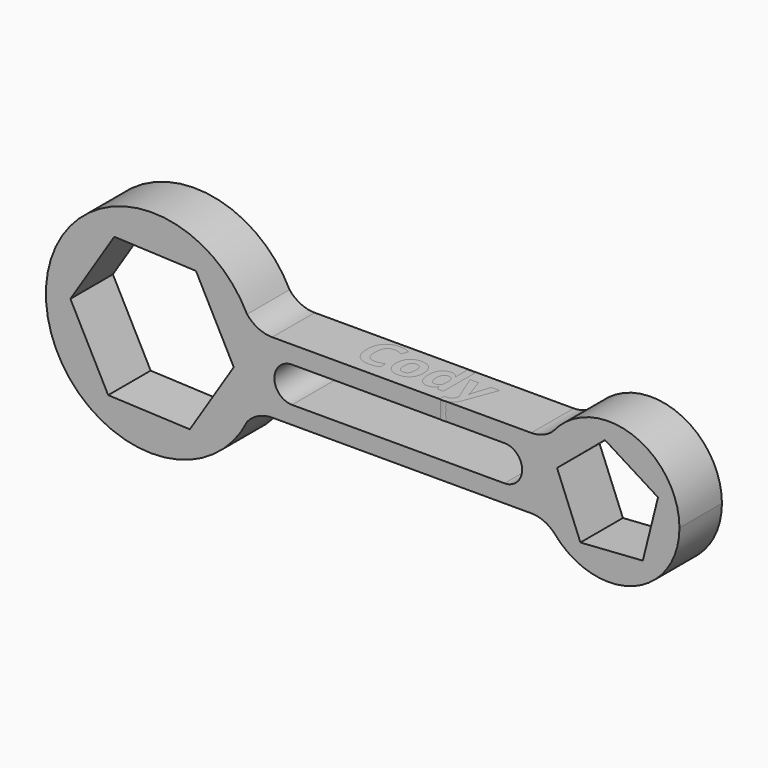
from build123d import *

# Parameters (mm, degrees)
F1_DEPTH     = 15
F2_TEXT_SIZE = 14.6601352349
F3_DEPTH     = 5


# Not quite as in the source:
# - Text() gives the source's letters only with a copy of the font that has no kerning and outlines rounded to 1/6400 em; it was checked with that copy


with BuildPart() as f1:
    # F0 (on Front) → F1 (new body)
    with BuildSketch(Plane.XZ):
        with BuildLine():
            ThreePointArc((-44.5868543681, -13.2794933275), (-42.2727545329, -6.8181696844), (-41.4876918451, 0))
            ThreePointArc((-41.4876918451, 0), (-42.2876779784, 6.8818013765), (-44.6449711908, 13.3965797082))
            ThreePointArc((-44.6449711908, 13.3965797082), (-101.4876206501, -0.065358216), (-44.5868543681, -13.2794933275))
        make_face()
        Polygon((-60.8156703444, -20.4802658777), (-83.8881116211, -19.4823746682), (-94.5601331218, 0.9978912095), (-82.1597133458, 20.4802658777), (-59.0872720691, 19.4823746682), (-48.4152505684, -0.9978912095), align=None, mode=Mode.SUBTRACT)
        with BuildLine():
            ThreePointArc((41.9423593748, 12.5529556275), (37.5154482696, -0.3543934672), (42.3969355922, -13.0967748813))
            ThreePointArc((42.3969355922, -13.0967748813), (64.5013191274, -18.7390961796), (77.5123081549, 0))
            ThreePointArc((77.5123081549, 0), (64.1681711492, 18.8599970255), (41.9423593748, 12.5529556275))
        make_face()
        Polygon((42.9262094907, 3.6496239321), (56.4759544087, 15), (71.4579049796, 5.6208858991), (67.1675147321, -11.5261014675), (49.5339571634, -12.7444083638), align=None, mode=Mode.SUBTRACT)
        with BuildLine():
            ThreePointArc((-44.6449711908, 13.3965797082), (-42.2876779784, 6.8818013765), (-41.4876918451, 0))
            ThreePointArc((-41.4876918451, 0), (-42.2727545329, -6.8181696844), (-44.5868543681, -13.2794933275))
            ThreePointArc((-44.5868543681, -13.2794933275), (-41.4324995346, -10.8601417529), (-37.551343441, -10))
            Line((-37.551343441, -10), (35.6224104762, -10))
            ThreePointArc((35.6224104762, -10), (39.3467965066, -10.8108939133), (42.3969355922, -13.0967748813))
            ThreePointArc((42.3969355922, -13.0967748813), (37.5154482696, -0.3543934672), (41.9423593748, 12.5529556275))
            ThreePointArc((41.9423593748, 12.5529556275), (39.0304647788, 10.6623457158), (35.6224104762, 10))
            Line((35.6224104762, 10), (-37.551343441, 10))
            ThreePointArc((-37.551343441, 10), (-41.4837825177, 10.8929262627), (-44.6449711908, 13.3965797082))
        make_face()
        with BuildLine():
            ThreePointArc((-31.9349189311, -5), (-36.9349189311, 0), (-31.9349189311, 5))
            Line((-31.9349189311, 5), (28.0650810689, 5))
            ThreePointArc((28.0650810689, 5), (33.0650810689, 0), (28.0650810689, -5))
            Line((28.0650810689, -5), (-31.9349189311, -5))
        make_face(mode=Mode.SUBTRACT)
    extrude(amount=F1_DEPTH)


with BuildPart() as f3:
    # F2 (on face) → F3 (new body)
    with BuildSketch(Plane.XY.offset(10)):
        with Locations((-18.492219504, -11.565955705)):
            Text('Cody', F2_TEXT_SIZE, font='Open Sans', font_style=FontStyle.BOLD, text_align=(TextAlign.LEFT, TextAlign.BOTTOM))
    extrude(amount=-F3_DEPTH)


solid = Compound([f1.part, f3.part])
